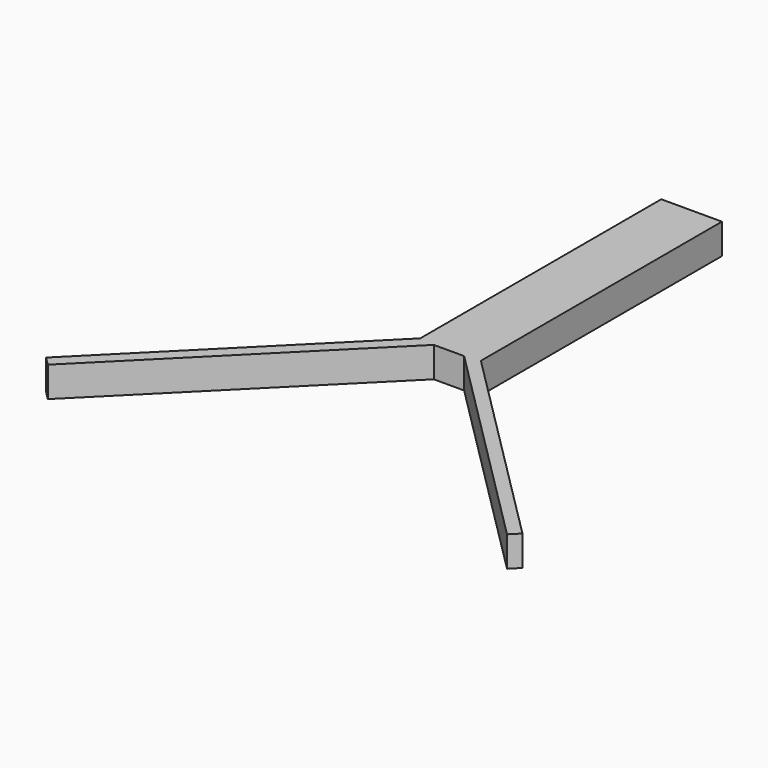
from build123d import *

# Parameters (mm, degrees)
F0_W     = 6.35
F0_H     = 63.5
F1_DEPTH = 6.35
F3_DEPTH = 6.35


# Not quite as in the source:
# - a feature names something its author has since deleted; it is built from what else it names


with BuildPart() as f1:
    # F0 (on Top) → F1 (new body)
    with BuildSketch(Plane.XY):
        with Locations((-3.175, -31.75)):
            Rectangle(F0_W, F0_H)
    extrude(amount=F1_DEPTH)

    # F2 (on face) → F3 (join)
    with BuildSketch(Plane(origin=(0, 0, 0), x_dir=(1, 0, 0), z_dir=(0, 0, -1))):
        Polygon((-4.9710512242, 61.7039487758), (-3.175, 63.5), (-48.0762806053, 108.4012806053), (-49.8723318296, 106.6052293811), align=None)
    extrude(amount=-F3_DEPTH)

    # F4: F1 across plane


with BuildPart() as f1_1:
    add(f1.part)
    add(f1.part.mirror(Plane.YZ))


solid = f1_1.part
